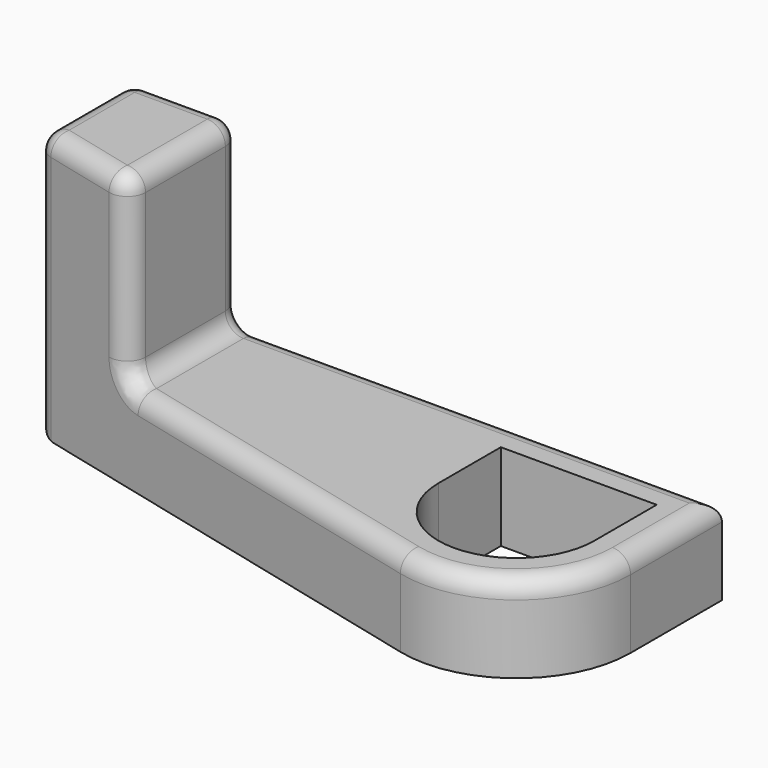
from build123d import *

# Parameters (mm, degrees)
F1_DEPTH = 24
F3_DEPTH = 50
F4_R     = 5


with BuildPart() as f1:
    # F0 (on Top) → F1 (new body)
    with BuildSketch(Plane.XY):
        with BuildLine():
            Line((-10, 0), (-10, 31.5))
            Line((-10, 31.5), (-110, 31.5))
            Line((-110, 31.5), (-110, 0))
            Line((-110, 0), (13.9543726236, -30.5828956689))
            ThreePointArc((13.9543726236, -30.5828956689), (-3.2985610707, -19.4237321033), (-10, 0))
        make_face()
        with BuildLine():
            Line((53, 31.5), (-10, 31.5))
            Line((-10, 31.5), (-10, 0))
            ThreePointArc((-10, 0), (-3.2985610707, -19.4237321033), (13.9543726236, -30.5828956689))
            ThreePointArc((13.9543726236, -30.5828956689), (40.9237321033, -24.7985610707), (53, 0))
            Line((53, 0), (53, 31.5))
        make_face()
        with BuildLine():
            ThreePointArc((43, 0), (21.5, -21.5), (0, 0))
            Line((0, 0), (0, 21.5))
            Line((0, 21.5), (43, 21.5))
            Line((43, 21.5), (43, 0))
        make_face(mode=Mode.SUBTRACT)
    extrude(amount=F1_DEPTH)

    # F2 (on face) → F3 (join)
    with BuildSketch(Plane.XY.offset(24)):
        Polygon((-80, -7.4018112524), (-80, 31.5), (-110, 31.5), (-110, 0), align=None)
    extrude(amount=F3_DEPTH)

    # F4
    f4_edges = [f1.edges().sort_by_distance(p)[0] for p in [
        (-110, 31.5, 37),
        (-110, 15.75, 74),
        (-110, 0, 37),
        (-110, 15.75, 0),
        (-80, 12.049094, 74),
        (-95, 31.5, 74),
        (-95, -3.700906, 74),
        (-80, -7.401811, 49),
        (-80, 31.5, 49),
        (-80, 12.049094, 24),
        (-13.5, 31.5, 24),
        (53, 15.75, 24),
        (40.923732, -24.798561, 24),
        (-33.022814, -18.992353, 24),
    ]]
    fillet(f4_edges, radius=F4_R)


solid = f1.part
